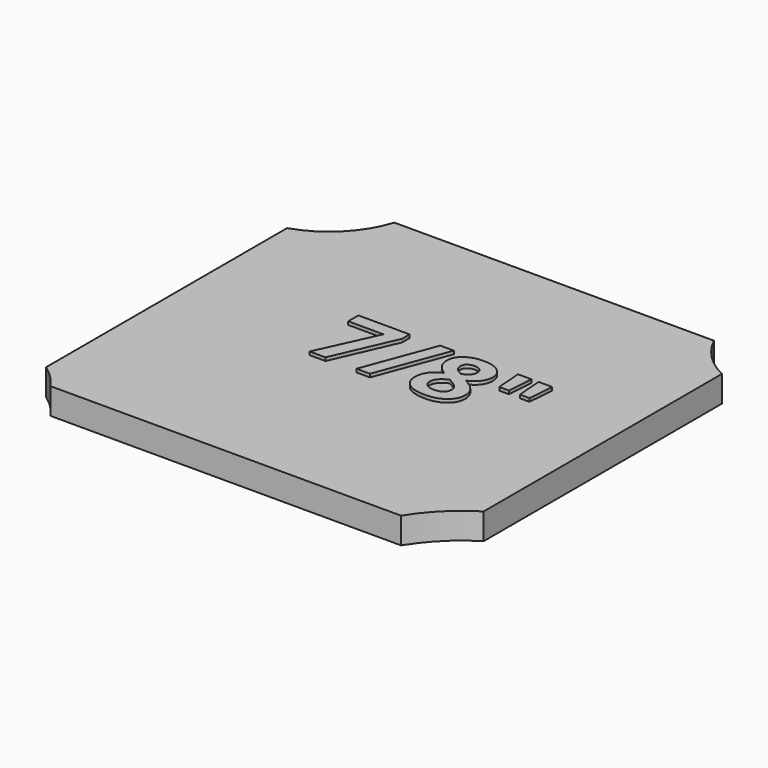
from build123d import *

# Parameters (mm, degrees)
F1_DEPTH     = 1.5875
F2_TEXT_SIZE = 12.132134806
F3_DEPTH     = 0.396875


# Not quite as in the source:
# - Text() gives the source's letters only with a copy of the font that has no kerning and outlines rounded to 1/6400 em; it was checked with that copy


with BuildPart() as f1:
    # F0 (on Top) → F1 (new body, symmetric)
    with BuildSketch(Plane.XY):
        with BuildLine():
            ThreePointArc((-79.3543815291, -31.2865550965), (-77.8466574232, -32.5483241919), (-76.5848883278, -34.0560482979))
            Line((-76.5848883278, -34.0560482979), (-34.1191226073, -34.0560482979))
            ThreePointArc((-34.1191226073, -34.0560482979), (-31.6613489008, -30.9490809262), (-28.5543815291, -28.4913072197))
            Line((-28.5543815291, -28.4913072197), (-28.5543815291, 6.0951293388))
            Line((-28.5543815291, 6.0951293388), (-28.5543815291, 7.5927037507))
            ThreePointArc((-28.5543815291, 7.5927037507), (-31.3938018407, 9.6057090272), (-33.4068071172, 12.4451293388))
            Line((-33.4068071172, 12.4451293388), (-34.9043815291, 12.4451293388))
            Line((-34.9043815291, 12.4451293388), (-72.1320317236, 12.4451293388))
            ThreePointArc((-72.1320317236, 12.4451293388), (-74.8642534686, 7.9550012782), (-79.3543815291, 5.2227795333))
            Line((-79.3543815291, 5.2227795333), (-79.3543815291, -31.2865550965))
        make_face()
    extrude(amount=F1_DEPTH, both=True)

    # F2 (on face) → F3 (join)
    with BuildSketch(Plane.XY.offset(1.5875)):
        with Locations((-62.7575293183, -13.7816863135)):
            Text('7/8"', F2_TEXT_SIZE, font='Open Sans', font_style=FontStyle.BOLD, text_align=(TextAlign.LEFT, TextAlign.BOTTOM))
    extrude(amount=F3_DEPTH)


solid = f1.part
